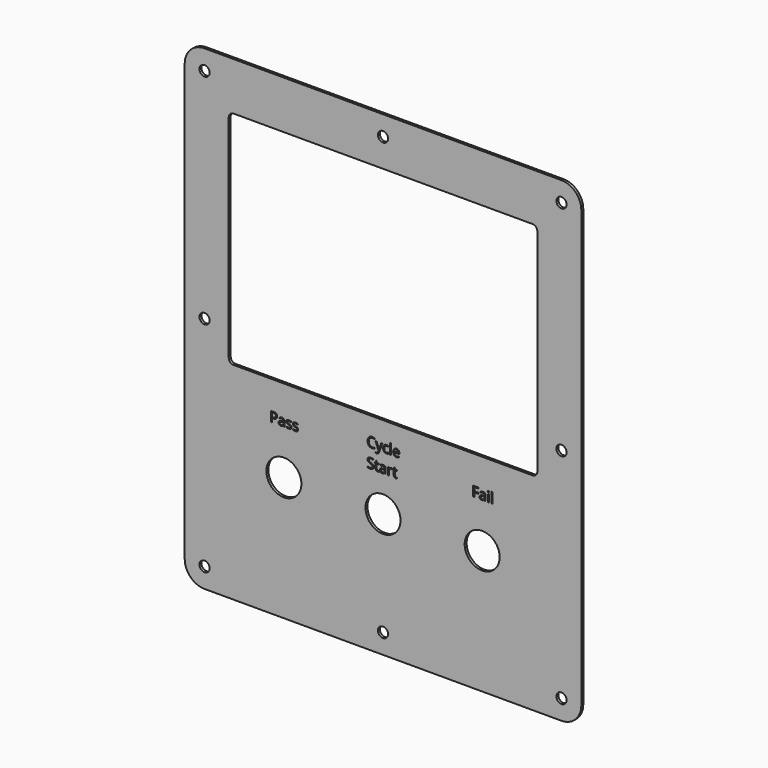
from build123d import *

# Parameters (mm, degrees)
F1_DEPTH      = 1.5875
F2_R          = 11.2141
F3_DEPTH      = 25.4
F5_DEPTH      = 25.4
F6_R          = 3.2639
F7_DEPTH      = 25.4
F8_TEXT_SIZE  = 8.8194444444
F9_TEXT_SIZE  = 8.8194444444
F10_TEXT_SIZE = 8.8194444444
F11_DEPTH     = 0.635


# Not quite as in the source:
# - Text() gives the source's letters only with a copy of the font that has no kerning and outlines rounded to 1/6400 em; it was checked with that copy


with BuildPart() as f1:
    # F0 (on Front) → F1 (new body)
    with BuildSketch(Plane.XZ):
        with BuildLine():
            Line((114.3, 152.4), (-114.3, 152.4))
            ThreePointArc((-114.3, 152.4), (-123.2802561211, 148.6802561211), (-127, 139.7))
            Line((-127, 139.7), (-127, -139.7))
            ThreePointArc((-127, -139.7), (-123.2802561211, -148.6802561211), (-114.3, -152.4))
            Line((-114.3, -152.4), (114.3, -152.4))
            ThreePointArc((114.3, -152.4), (123.2802561211, -148.6802561211), (127, -139.7))
            Line((127, -139.7), (127, 139.7))
            ThreePointArc((127, 139.7), (123.2802561211, 148.6802561211), (114.3, 152.4))
        make_face()
    extrude(amount=F1_DEPTH)

    # F2 (on face) → F3 (cut)
    with BuildSketch(Plane.XZ.offset(1.5875)):
        with Locations((-63.5, -73.025)):
            Circle(F2_R)
        with Locations((0, -73.025)):
            Circle(F2_R)
        with Locations((63.5, -73.025)):
            Circle(F2_R)
    extrude(amount=-F3_DEPTH, mode=Mode.SUBTRACT)

    # F4 (on face) → F5 (cut)
    with BuildSketch(Plane.XZ.offset(1.5875)):
        with BuildLine():
            ThreePointArc((98.806, 118.618), (97.9132614691, 120.7732614691), (95.758, 121.666))
            Line((95.758, 121.666), (-95.758, 121.666))
            ThreePointArc((-95.758, 121.666), (-97.9132614691, 120.7732614691), (-98.806, 118.618))
            Line((-98.806, 118.618), (-98.806, -17.018))
            ThreePointArc((-98.806, -17.018), (-97.9132614691, -19.1732614691), (-95.758, -20.066))
            Line((-95.758, -20.066), (95.758, -20.066))
            ThreePointArc((95.758, -20.066), (97.9132614691, -19.1732614691), (98.806, -17.018))
            Line((98.806, -17.018), (98.806, 118.618))
        make_face()
    extrude(amount=-F5_DEPTH, mode=Mode.SUBTRACT)

    # F6 (on face) → F7 (cut)
    with BuildSketch(Plane.XZ.offset(1.5875)):
        with Locations((-114.3, 139.7)):
            Circle(F6_R)
        with Locations((-114.3, 0)):
            Circle(F6_R)
        with Locations((-114.3, -139.7)):
            Circle(F6_R)
        with Locations((0, 139.7)):
            Circle(F6_R)
        Circle(F6_R)
        with Locations((0, -139.7)):
            Circle(F6_R)
        with Locations((114.3, 139.7)):
            Circle(F6_R)
        with Locations((114.3, 0)):
            Circle(F6_R)
        with Locations((114.3, -139.7)):
            Circle(F6_R)
    extrude(amount=-F7_DEPTH, mode=Mode.SUBTRACT)

    # F8 (on face) + F9 (on face) + F10 (on face) → F11 (cut)
    with BuildSketch(Plane.XZ.offset(1.5875)):
        with Locations((-72.6115885417, -44.45)):
            Text('Pass', F8_TEXT_SIZE, font='Open Sans', text_align=(TextAlign.LEFT, TextAlign.BOTTOM))
    with BuildSketch(Plane.XZ.offset(1.5875)):
        with Locations((-10.4069881564, -38.1)):
            Text('Cycle', F9_TEXT_SIZE, font='Open Sans', text_align=(TextAlign.LEFT, TextAlign.BOTTOM))
        with Locations((-10.4069881564, -50.0944444444)):
            Text('Start', F9_TEXT_SIZE, font='Open Sans', text_align=(TextAlign.LEFT, TextAlign.BOTTOM))
    with BuildSketch(Plane.XZ.offset(1.5875)):
        with Locations((56.9198676215, -44.45)):
            Text('Fail', F10_TEXT_SIZE, font='Open Sans', text_align=(TextAlign.LEFT, TextAlign.BOTTOM))
    extrude(amount=-F11_DEPTH, mode=Mode.SUBTRACT)


solid = f1.part
